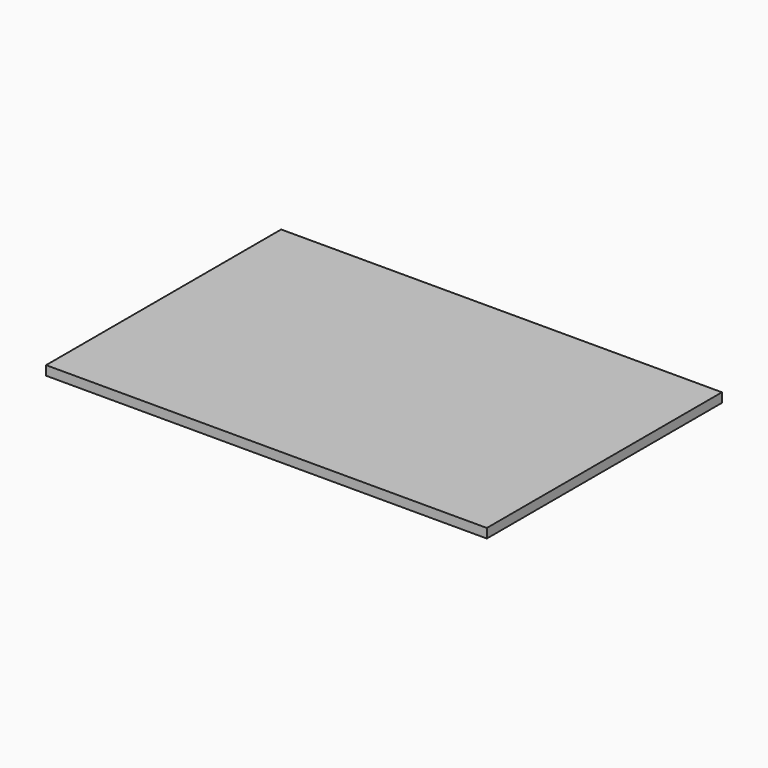
from build123d import *

# Parameters (mm, degrees)
F1_DEPTH = 3.175


# Not quite as in the source:
# - a length typed as a fraction of an inch, garbled in the dataset ("3 / 203.2 mm" for 3/8 in), is restored


with BuildPart() as f1:
    # F0 (on Top) → F1 (new body, symmetric)
    with BuildSketch(Plane.XY):
        Polygon((154.0753036737, -163.6231148611), (-145.9246963263, 36.3768851389), (-145.9246963263, -163.6231148611), align=None)
        Polygon((154.0753036737, 36.3768851389), (-145.9246963263, 36.3768851389), (154.0753036737, -163.6231148611), align=None)
    extrude(amount=F1_DEPTH, both=True)


solid = f1.part
